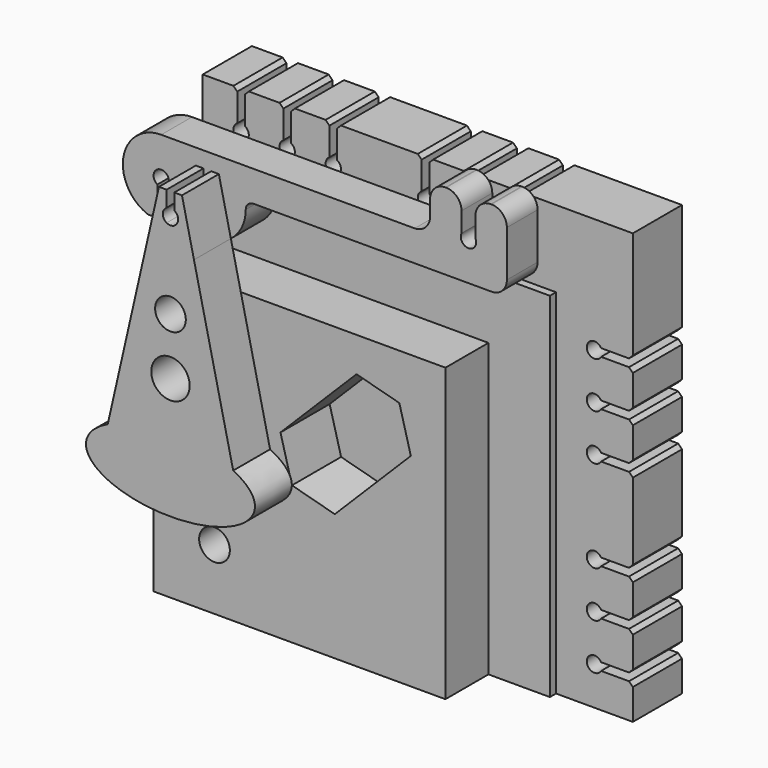
from build123d import *

# Parameters (mm, degrees)
F5_DEPTH     = 8
F6_DEPTH     = 1
F7_DEPTH     = 8
F8_SIZE      = 0.5
F9_D         = 2.5
F13_DEPTH    = 8
F15_DEPTH    = 5
F16_T1_DEPTH = 5
F16_T3_DEPTH = 12.0818393869
F16_T5_DEPTH = 10
F17_D        = 4
F18_R        = 2
F19_R        = 2.5
F19_R_2      = 2
F20_DEPTH    = 6


# Not quite as in the source:
# - a fillet or chamfer that OpenCascade refuses, or shapes differently, is made with other operations: its cross-section is extruded or revolved along the edge and cut away or added
# - a feature names something its author has since deleted; it is built from what else it names


with BuildPart() as f5:
    # F3 (on Front) → F5 (new body)
    with BuildSketch(Plane.XZ):
        Polygon((0, 38), (0, 0), (38, 38), align=None)
        Polygon((0, 46), (0, 38), (38, 38), (46, 46), align=None)
        Polygon((46, 46), (56, 56), (0, 56), (0, 46), align=None)
    extrude(amount=-F5_DEPTH)

    # F4 (on Front) → F7 (cut, through all)
    with BuildSketch(Plane.XZ):
        with BuildLine():
            ThreePointArc((4.5, 51.8660254038), (4.5, 50.1339745962), (6, 51))
            ThreePointArc((6, 51), (5.8660254038, 51.5), (5.5, 51.8660254038))
            ThreePointArc((5.5, 51.8660254038), (5, 52), (4.5, 51.8660254038))
        make_face()
        with BuildLine():
            ThreePointArc((4.5, 51.8660254038), (5, 52), (5.5, 51.8660254038))
            Line((5.5, 51.8660254038), (5.5, 56))
            Line((5.5, 56), (4.5, 56))
            Line((4.5, 56), (4.5, 51.8660254038))
        make_face()
        with BuildLine():
            ThreePointArc((10.5, 51.8660254038), (10.5, 50.1339745962), (12, 51))
            ThreePointArc((12, 51), (11.8660254038, 51.5), (11.5, 51.8660254038))
            ThreePointArc((11.5, 51.8660254038), (11, 52), (10.5, 51.8660254038))
        make_face()
        with BuildLine():
            ThreePointArc((10.5, 51.8660254038), (11, 52), (11.5, 51.8660254038))
            Line((11.5, 51.8660254038), (11.5, 56))
            Line((11.5, 56), (10.5, 56))
            Line((10.5, 56), (10.5, 51.8660254038))
        make_face()
        with BuildLine():
            ThreePointArc((28.5, 51.8660254038), (28.5, 50.1339745962), (30, 51))
            ThreePointArc((30, 51), (29.8660254038, 51.5), (29.5, 51.8660254038))
            ThreePointArc((29.5, 51.8660254038), (29, 52), (28.5, 51.8660254038))
        make_face()
        with BuildLine():
            ThreePointArc((28.5, 51.8660254038), (29, 52), (29.5, 51.8660254038))
            Line((29.5, 51.8660254038), (29.5, 56))
            Line((29.5, 56), (28.5, 56))
            Line((28.5, 56), (28.5, 51.8660254038))
        make_face()
        with BuildLine():
            ThreePointArc((34.5, 51.8660254038), (34.5, 50.1339745962), (36, 51))
            ThreePointArc((36, 51), (35.8660254038, 51.5), (35.5, 51.8660254038))
            ThreePointArc((35.5, 51.8660254038), (35, 52), (34.5, 51.8660254038))
        make_face()
        with BuildLine():
            ThreePointArc((34.5, 51.8660254038), (35, 52), (35.5, 51.8660254038))
            Line((35.5, 51.8660254038), (35.5, 56))
            Line((35.5, 56), (34.5, 56))
            Line((34.5, 56), (34.5, 51.8660254038))
        make_face()
        with BuildLine():
            ThreePointArc((40.5, 51.8660254038), (40.5, 50.1339745962), (42, 51))
            ThreePointArc((42, 51), (41.8660254038, 51.5), (41.5, 51.8660254038))
            ThreePointArc((41.5, 51.8660254038), (41, 52), (40.5, 51.8660254038))
        make_face()
        with BuildLine():
            ThreePointArc((40.5, 51.8660254038), (41, 52), (41.5, 51.8660254038))
            Line((41.5, 51.8660254038), (41.5, 56))
            Line((41.5, 56), (40.5, 56))
            Line((40.5, 56), (40.5, 51.8660254038))
        make_face()
        with BuildLine():
            ThreePointArc((16.5, 51.8660254038), (17, 52), (17.5, 51.8660254038))
            Line((17.5, 51.8660254038), (17.5, 56))
            Line((17.5, 56), (16.5, 56))
            Line((16.5, 56), (16.5, 51.8660254038))
        make_face()
        with BuildLine():
            ThreePointArc((16.5, 51.8660254038), (16.5, 50.1339745962), (18, 51))
            ThreePointArc((18, 51), (17.8660254038, 51.5), (17.5, 51.8660254038))
            ThreePointArc((17.5, 51.8660254038), (17, 52), (16.5, 51.8660254038))
        make_face()
    extrude(amount=-F7_DEPTH, mode=Mode.SUBTRACT)

    # F8
    f8_edges = [f5.edges().sort_by_distance(p)[0] for p in [
        (4.5, 4, 56),
        (5.5, 4, 56),
        (10.5, 4, 56),
        (11.5, 4, 56),
        (40.5, 4, 56),
        (41.5, 4, 56),
        (35.5, 4, 56),
        (34.5, 4, 56),
        (29.5, 4, 56),
        (28.5, 4, 56),
        (16.5, 4, 56),
        (17.5, 4, 56),
    ]]
    chamfer(f8_edges, length=F8_SIZE)

    # F9 (through all)
    with Locations(Plane.XZ):
        with Locations((10, 42), (26, 42)):
            Hole(F9_D / 2)

    # F10: F5 across face


with BuildPart() as f6:
    # F3 (on Front) → F6 (new body)
    with BuildSketch(Plane.XZ):
        Polygon((0, 46), (0, 38), (38, 38), (46, 46), align=None)
    extrude(amount=F6_DEPTH)

    # F11: F6 across face


with BuildPart() as f5_1:
    add(f5.part)
    add(f5.part.mirror(Plane(origin=(28, 4, 28), x_dir=(0, 1, 0), z_dir=(0.7071067812, 0, -0.7071067812))))


with BuildPart() as f6_1:
    add(f6.part)
    add(f6.part.mirror(Plane(origin=(42, -0.5, 42), x_dir=(0, 1, 0), z_dir=(0.7071067812, 0, -0.7071067812))))


with BuildPart() as f13:
    # F12 (on face) → F13 (new body)
    with BuildSketch(Plane.XZ):
        Polygon((38, 38), (0, 38), (0, 0), (18.0180221587, 18.0180221587), (16.5237297051, 23.594797517), (26.4232246417, 33.4942924536), (32, 32), align=None)
        Polygon((38, 0), (38, 38), (32, 32), (33.4942924536, 26.4232246417), (23.594797517, 16.5237297051), (18.0180221587, 18.0180221587), (0, 0), align=None)
    extrude(amount=F13_DEPTH)

    # F17 (through all)
    with Locations(Plane(origin=(0, 0, 0), x_dir=(1, 0, 0), z_dir=(0, 1, 0))):
        with Locations((7.9334294423, -7.9334294423)):
            Hole(F17_D / 2)


with BuildPart() as f15:
    # F14 (on face) → F15 (new body)
    with BuildSketch(Plane.XZ.offset(8)):
        with BuildLine():
            ThreePointArc((8, 47), (6.527864045, 48.7639320225), (6, 51))
            ThreePointArc((6, 51), (5.8660254038, 50.5), (5.5, 50.1339745962))
            Line((5.5, 50.1339745962), (5.5, 46.0250628145))
            ThreePointArc((5.5, 46.0250628145), (6.8166247904, 46.3416876048), (8, 47))
        make_face()
        with BuildLine():
            ThreePointArc((4.5, 50.1339745962), (4.5, 51.8660254038), (6, 51))
            ThreePointArc((6, 51), (6.527864045, 53.2360679775), (8, 55))
            ThreePointArc((8, 55), (6.5811388301, 55.7434164903), (5, 56))
            ThreePointArc((5, 56), (0.0062696344, 51.2503138753), (4.5, 46.0250628145))
            Line((4.5, 46.0250628145), (4.5, 50.1339745962))
        make_face()
        with BuildLine():
            ThreePointArc((8, 55), (6.527864045, 53.2360679775), (6, 51))
            ThreePointArc((6, 51), (6.527864045, 48.7639320225), (8, 47))
            ThreePointArc((8, 47), (9.472135955, 48.7639320225), (10, 51))
            ThreePointArc((10, 51), (9.472135955, 53.2360679775), (8, 55))
        make_face()
        with BuildLine():
            ThreePointArc((5, 56), (6.5811388301, 55.7434164903), (8, 55))
            ThreePointArc((8, 55), (9.4188611699, 55.7434164903), (11, 56))
            Line((11, 56), (5, 56))
        make_face()
        with BuildLine():
            ThreePointArc((11, 56), (9.4188611699, 55.7434164903), (8, 55))
            ThreePointArc((8, 55), (9.472135955, 53.2360679775), (10, 51))
            ThreePointArc((10, 51), (11, 52), (12, 51))
            ThreePointArc((12, 51), (11.8660254038, 50.5), (11.5, 50.1339745962))
            Line((11.5, 50.1339745962), (11.5, 46.0250628145))
            ThreePointArc((11.5, 46.0250628145), (14.7080992435, 47.6458980338), (16, 51))
            ThreePointArc((16, 51), (15.974680765, 51.50254481), (15.8989794856, 52))
            ThreePointArc((15.8989794856, 52), (14.1622776602, 54.8729833462), (11, 56))
        make_face()
        with BuildLine():
            ThreePointArc((10, 51), (9.472135955, 48.7639320225), (8, 47))
            ThreePointArc((8, 47), (9.1833752096, 46.3416876048), (10.5, 46.0250628145))
            Line((10.5, 46.0250628145), (10.5, 50.1339745962))
            ThreePointArc((10.5, 50.1339745962), (10.1339745962, 50.5), (10, 51))
        make_face()
        with BuildLine():
            ThreePointArc((10.5, 46.0250628145), (9.1833752096, 46.3416876048), (8, 47))
            ThreePointArc((8, 47), (6.8166247904, 46.3416876048), (5.5, 46.0250628145))
            Line((5.5, 46.0250628145), (10.5, 46.0250628145))
        make_face()
        with BuildLine():
            Line((40, 56), (11, 56))
            ThreePointArc((11, 56), (14.1622776602, 54.8729833462), (15.8989794856, 52))
            Line((15.8989794856, 52), (41, 52))
            Line((41, 52), (50, 52))
            Line((50, 52), (50, 62))
            Line((50, 62), (45.9, 62))
            Line((45.9, 62), (45.9, 57.4358898944))
            ThreePointArc((45.9, 57.4358898944), (45.9746794345, 57.2236067977), (46, 57))
            ThreePointArc((46, 57), (44.7763932023, 56.0253205655), (44.1, 57.4358898944))
            Line((44.1, 57.4358898944), (44.1, 62))
            Line((44.1, 62), (40, 62))
            Line((40, 62), (40, 56))
        make_face()
    extrude(amount=F15_DEPTH)

    # F16: fillet of radius 1 on 5 edges, made by hand

    # F16_s2 → F16_t1 (join)
    with BuildSketch(Plane.XZ.offset(8)):
        with BuildLine():
            ThreePointArc((16, 51), (16.2928932188, 51.7071067812), (17, 52))
            Line((17, 52), (15.8989794856, 52))
            ThreePointArc((15.8989794856, 52), (15.974680765, 51.50254481), (16, 51))
        make_face()
    extrude(amount=F16_T1_DEPTH)

    # F16_s4 → F16_t3 (cut)
    with BuildSketch(Plane.XZ.offset(4.4590803066)):
        with BuildLine():
            ThreePointArc((4.5, 47.2919007565), (4.0590169944, 46.4627445589), (3.125, 46.3648759456))
            ThreePointArc((3.125, 46.3648759456), (3.8004065309, 46.1460350734), (4.5, 46.0250628145))
            Line((4.5, 46.0250628145), (4.5, 47.2919007565))
        make_face()
        with BuildLine():
            ThreePointArc((11.5, 47.2919007565), (11.9409830056, 46.4627445589), (12.875, 46.3648759456))
            ThreePointArc((12.875, 46.3648759456), (12.1995934691, 46.1460350734), (11.5, 46.0250628145))
            Line((11.5, 46.0250628145), (11.5, 47.2919007565))
        make_face()
    extrude(amount=F16_T3_DEPTH, mode=Mode.SUBTRACT)

    # F16_s6 → F16_t5 (cut)
    with BuildSketch(Plane.XZ.offset(5.5)):
        with BuildLine():
            ThreePointArc((5.5, 47.0250628145), (5.7928932188, 46.3179560333), (6.5, 46.0250628145))
            Line((6.5, 46.0250628145), (5.5, 46.0250628145))
            Line((5.5, 46.0250628145), (5.5, 47.0250628145))
        make_face()
        with BuildLine():
            ThreePointArc((9.5, 46.0250628145), (10.2071067812, 46.3179560333), (10.5, 47.0250628145))
            Line((10.5, 47.0250628145), (10.5, 46.0250628145))
            Line((10.5, 46.0250628145), (9.5, 46.0250628145))
        make_face()
    extrude(amount=F16_T5_DEPTH, mode=Mode.SUBTRACT)

    # F18
    f18_edges = [f15.edges().sort_by_distance(p)[0] for p in [
        (40, -10.5, 56),
        (40, -10.5, 62),
        (44.1, -10.5, 62),
        (45.9, -10.5, 62),
        (50, -10.5, 62),
        (50, -10.5, 52),
    ]]
    fillet(f18_edges, radius=F18_R)


with BuildPart() as f20:
    # F19 (on face) → F20 (new body)
    with BuildSketch(Plane.XZ.offset(13)):
        with BuildLine():
            Line((10.5, 51.8660254038), (10.5, 53.9330127019))
            Line((10.5, 53.9330127019), (9.5, 53.9330127019))
            Line((9.5, 53.9330127019), (7.7055859223, 46.0250628145))
            Line((7.7055859223, 46.0250628145), (9.5, 46.0250628145))
            ThreePointArc((9.5, 46.0250628145), (10.2071067812, 46.3179560333), (10.5, 47.0250628145))
            Line((10.5, 47.0250628145), (10.5, 50.1339745962))
            ThreePointArc((10.5, 50.1339745962), (10, 51), (10.5, 51.8660254038))
        make_face()
        with BuildLine():
            Line((12.5, 53.9330127019), (11.5, 53.9330127019))
            Line((11.5, 53.9330127019), (11.5, 51.8660254038))
            ThreePointArc((11.5, 51.8660254038), (11.8660254038, 51.5), (12, 51))
            ThreePointArc((12, 51), (11.8660254038, 50.5), (11.5, 50.1339745962))
            Line((11.5, 50.1339745962), (11.5, 47.2919007565))
            ThreePointArc((11.5, 47.2919007565), (11.9409830056, 46.4627445589), (12.875, 46.3648759456))
            ThreePointArc((12.875, 46.3648759456), (13.4921846161, 46.6653701612), (14.0623951785, 47.0475658423))
            Line((14.0623951785, 47.0475658423), (12.5, 53.9330127019))
        make_face()
        with BuildLine():
            ThreePointArc((11.5, 50.1339745962), (11, 50), (10.5, 50.1339745962))
            Line((10.5, 50.1339745962), (10.5, 47.0250628145))
            ThreePointArc((10.5, 47.0250628145), (10.2071067812, 46.3179560333), (9.5, 46.0250628145))
            Line((9.5, 46.0250628145), (7.7055859223, 46.0250628145))
            Line((7.7055859223, 46.0250628145), (2.8331882585, 24.5524957869))
            add(Edge.make_bspline(
                [(19.1668117415, 24.5524957869), (11, 28.4625329607), (2.8331882585, 24.5524957869)],
                knots=[3.8756875041, 3.8756875041, 3.8756875041, 5.5490904567, 5.5490904567, 5.5490904567], degree=2, weights=[1, 0.6699154133, 1]))
            Line((19.1668117415, 24.5524957869), (14.0623951785, 47.0475658423))
            ThreePointArc((14.0623951785, 47.0475658423), (13.4921846161, 46.6653701612), (12.875, 46.3648759456))
            ThreePointArc((12.875, 46.3648759456), (11.9409830056, 46.4627445589), (11.5, 47.2919007565))
            Line((11.5, 47.2919007565), (11.5, 50.1339745962))
        make_face()
        with Locations((11, 32.4375927448)):
            Circle(F19_R, mode=Mode.SUBTRACT)
        with Locations((11, 39.8379452527)):
            Circle(F19_R_2, mode=Mode.SUBTRACT)
        with BuildLine():
            add(Edge.make_bspline(
                [(19.1668117415, 24.5524957869), (11, 28.4625329607), (2.8331882585, 24.5524957869)],
                knots=[3.8756875041, 3.8756875041, 3.8756875041, 5.5490904567, 5.5490904567, 5.5490904567], degree=2, weights=[1, 0.6699154133, 1]))
            add(Edge.make_bspline(
                [(2.8331882585, 24.5524957869), (0, 23.1960458329), (0, 21.3690232486)],
                knots=[5.5490904567, 5.5490904567, 5.5490904567, 6.2831853072, 6.2831853072, 6.2831853072], degree=2, weights=[1, 0.9333909768, 1]))
            add(Edge.make_bspline(
                [(0, 21.3690232486), (0, 14.4508313592), (14.9474720292, 16.9335012661), (29.8949440584, 19.416171173), (19.1668117415, 24.5524957869)],
                knots=[0, 0, 0, 1.9378437521, 1.9378437521, 3.8756875041, 3.8756875041, 3.8756875041], degree=2, weights=[1, 0.5661885315, 1, 0.5661885315, 1]))
        make_face()
    extrude(amount=F20_DEPTH)


solid = Compound([f5_1.part, f6_1.part, f13.part, f15.part, f20.part])
